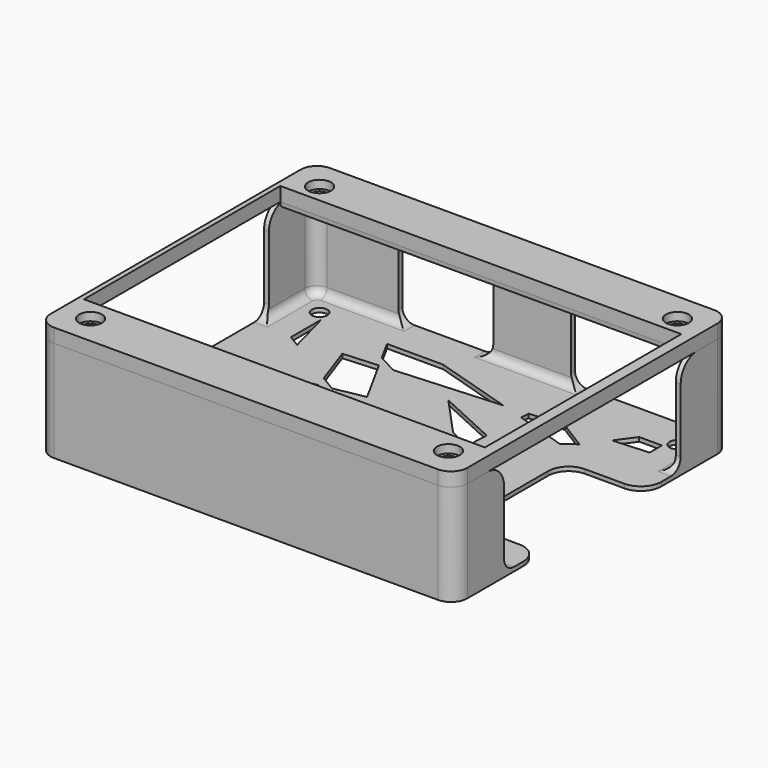
from build123d import *

# Parameters (mm, degrees)
F1_W      = 101.8573045731
F1_H      = 84.3658432415
F1_W_2    = 99.4573066576
F1_H_2    = 81.9658453261
F2_DEPTH  = 1
F3_DEPTH  = 23.7
F4_W      = 54
F4_H      = 23.7
F5_DEPTH  = 101.8583045731
F7_DEPTH  = 25
F0_R      = 1.9
F8_DEPTH  = 25
F9_R      = 3
F10_R     = 4
F11_R     = 3
F12_R     = 5
F14_DEPTH = 25
F15_R     = 5
F17_R     = 1.9
F18_DEPTH = 3.4
F19_DEPTH = 1
F19_TAPER = 4
F20_R     = 2.8028286172
F20_R_2   = 1.9
F21_DEPTH = 2
F23_DEPTH = 25
F24_R     = 2


with BuildPart() as f2:
    # F1 (on Top) → F2 (new body)
    with BuildSketch(Plane.XY):
        Rectangle(F1_W, F1_H)
        Rectangle(F1_W_2, F1_H_2, mode=Mode.SUBTRACT)
        Rectangle(F1_W_2, F1_H_2)
    extrude(amount=-F2_DEPTH)

    # F1 (on Top) → F3 (join)
    with BuildSketch(Plane.XY):
        Rectangle(F1_W, F1_H)
        Rectangle(F1_W_2, F1_H_2, mode=Mode.SUBTRACT)
    extrude(amount=F3_DEPTH)

    # F4 (on face) → F5 (cut, through all)
    with BuildSketch(Plane(origin=(-50.9286522865, 0, 0), x_dir=(0, -1, 0), z_dir=(-1, 0, 0))):
        with Locations((0, 11.85)):
            Rectangle(F4_W, F4_H)
    extrude(amount=-F5_DEPTH, mode=Mode.SUBTRACT)

    # F6 (on face) → F7 (cut)
    with BuildSketch(Plane(origin=(0, 42.1829216208, 0), x_dir=(-1, 0, 0), z_dir=(0, 1, 0))):
        Polygon((-12.9286522865, 0), (-12.9286522865, 11.35), (-12.9286522865, 25.37307702), (-44.0330952406, 25.37307702), (-44.0330952406, 0), align=None)
        Polygon((6.0713477135, 25.847222656), (6.0713477135, 7.5958021916), (6.0713477135, 0), (29.2794182897, 0), (29.2794182897, 25.847222656), align=None)
    extrude(amount=-F7_DEPTH, mode=Mode.SUBTRACT)

    # F0 (on Top) → F8 (cut)
    with BuildSketch(Plane.XY):
        with Locations((43.7286533288, 34.982922663)):
            Circle(F0_R)
        with Locations((43.7286533288, -34.982922663)):
            Circle(F0_R)
        with Locations((-43.7286533288, 34.982922663)):
            Circle(F0_R)
        with Locations((-43.7286533288, -34.982922663)):
            Circle(F0_R)
    extrude(amount=-F8_DEPTH, mode=Mode.SUBTRACT)

    # F9
    f9_edges = [f2.edges().sort_by_distance(p)[0] for p in [
        (49.728653, -40.982923, 11.85),
        (-49.728653, -40.982923, 11.85),
        (-49.728653, 40.982923, 11.85),
        (49.728653, 40.982923, 11.85),
    ]]
    fillet(f9_edges, radius=F9_R)

    # F10
    f10_edges = [f2.edges().sort_by_distance(p)[0] for p in [
        (-50.928652, 42.182922, 11.35),
        (-50.928652, -42.182922, 11.35),
        (50.928652, -42.182922, 11.35),
        (50.928652, 42.182922, 11.35),
    ]]
    fillet(f10_edges, radius=F10_R)

    # F11
    f11_edges = [f2.edges().sort_by_distance(p)[0] for p in [
        (-50.328653, 27, 0),
        (-29.279418, 41.582922, 0),
        (-6.071348, 41.582922, 0),
        (12.928652, 41.582922, 0),
        (44.033095, 41.582922, 0),
        (50.328653, 27, 0),
        (50.328653, -27, 0),
        (-50.328653, -27, 0),
    ]]
    fillet(f11_edges, radius=F11_R)

    # F12
    f12_edges = [f2.edges().sort_by_distance(p)[0] for p in [
        (50.328653, -27, 23.7),
        (50.328653, 27, 23.7),
        (44.033095, 41.582922, 23.7),
        (12.928652, 41.582922, 23.7),
        (-6.071348, 41.582922, 23.7),
        (-29.279418, 41.582922, 23.7),
        (-50.328653, 27, 23.7),
        (-50.328653, -27, 23.7),
    ]]
    fillet(f12_edges, radius=F12_R)

    # F13 (on face) → F14 (cut)
    with BuildSketch(Plane(origin=(0, 0, -1), x_dir=(1, 0, 0), z_dir=(0, 0, -1))):
        Polygon((50.9286522865, 0), (50.9286522865, 16.0555634648), (31.2976017594, 16.0555634648), (31.2976017594, 0), (31.2976017594, -16.0555634648), (50.9286522865, -16.0555634648), align=None)
    extrude(amount=-F14_DEPTH, mode=Mode.SUBTRACT)

    # F15
    f15_edges = [f2.edges().sort_by_distance(p)[0] for p in [
        (50.928652, -16.055563, -0.5),
        (50.928652, 16.055563, -0.5),
        (31.297602, -16.055563, -0.5),
        (31.297602, 16.055563, -0.5),
    ]]
    fillet(f15_edges, radius=F15_R)

    # F22 (on face) → F23 (cut)
    with BuildSketch(Plane(origin=(0, 0, -1), x_dir=(1, 0, 0), z_dir=(0, 0, -1))):
        Polygon((-29.4763375006, 14.8269218376), (-41.6286520634, 12.3842693865), (-30.3887994705, 9.3961659471), (-29.0076859915, 14.5912712147), align=None)
        Polygon((-10.8715390327, 29.0833591801), (-15.9313136106, 27.743293622), (-12.1721135632, 25.3909763414), align=None)
        Polygon((-24.1448692977, 32.8829213977), (-41.6286520634, 32.8829213977), (-41.6286520634, 20.9374334663), (-26.2368387197, 25.013907353), align=None)
        Polygon((-15.6970236635, 15.3836163194), (-20.9847782869, 10.5571367647), (-17.9368811333, 9.0245718443), align=None)
        Polygon((-32.9943795181, -0.4048119131), (-35.4038891191, -9.468264128), (-25.1375269952, -11.4183482529), (-18.8833677873, 6.3374585753), (-24.0909853022, 7.7218984226), align=None)
        Polygon((-26.1431570385, -14.2733719574), (-29.7097056452, -24.3989453556), (-21.2132293912, -24.9611379018), (-14.8402038289, -13.3743133936), (-22.301487185, -11.9570508766), align=None)
        Polygon((-5.5360004898, 2.789074484), (-5.8971521934, 2.885086299), (-9.9716865757, -4.5228417533), (-1.342161859, 0.6802992716), align=None)
        Polygon((-22.7277484281, -27.7146913158), (-25.5703963339, -32.8829213977), (-9.9331525483, -25.70751498), (-17.8456036869, -25.18396605), align=None)
        Polygon((-39.206147282, -23.77058737), (-41.6286520634, -23.6102957278), (-41.6286520634, -32.8829213977), align=None)
        Polygon((-38.6929646651, -21.840233524), (-41.6286520634, -23.6102957278), (-39.206147282, -23.77058737), align=None)
        Polygon((-9.9331525483, -25.70751498), (-25.5703963339, -32.8829213977), (-11.849696748, -32.8829213977), (-5.5335982145, -25.9986235031), align=None)
        Polygon((-5.5335982145, -25.9986235031), (-11.849696748, -32.8829213977), (7.6651824891, -26.8719568602), align=None)
        Polygon((2.9486668234, -16.7532896893), (-1.8734205455, -22.0091744329), (7.6390471274, -17.6442222378), align=None)
        Polygon((7.0570029567, -12.2753655968), (2.9486668234, -16.7532896893), (7.6390471274, -17.6442222378), (12.9477911078, -15.2082177764), (12.6630292841, -9.3694065932), align=None)
        with BuildLine():
            Line((13.4300364537, -25.0962690722), (13.5355816391, -27.2603878458))
            Line((13.5355816391, -27.2603878458), (21.9606679178, -27.8178566794))
            Line((21.9606679178, -27.8178566794), (29.0744918276, -23.3972282347))
            ThreePointArc((29.0744918276, -23.3972282347), (27.5588064071, -22.3747269573), (26.1859746307, -21.1671905935))
            Line((26.1859746307, -21.1671905935), (13.4300364537, -25.0962690722))
        make_face()
        Polygon((32.8745938929, -28.5400063859), (36.0836610198, -32.8829213977), (41.6286520634, -29.1192425428), align=None)
        Polygon((41.6286520634, -29.1192425428), (36.0836610198, -32.8829213977), (41.6286520634, -32.8829213977), align=None)
        Polygon((1.7053230027, 16.7071783437), (4.4184203361, 21.6398719863), (-3.6014076253, 20.0278620004), align=None)
        Polygon((11.0853349082, 22.9799422369), (4.4184203361, 21.6398719863), (1.7053230027, 16.7071783437), (11.6961624804, 10.4554162521), align=None)
        Polygon((27.8325551851, 26.3461848112), (15.948086977, 32.8829213977), (19.0470213151, 24.5802655922), align=None)
        with BuildLine():
            ThreePointArc((21.9976015364, 11.0555634648), (22.1447687516, 13.1018587106), (22.5832412801, 15.1060354155))
            Line((22.5832412801, 15.1060354155), (13.2536724335, 9.4808052893))
            Line((13.2536724335, 9.4808052893), (21.9976015364, 4.0092966519))
            Line((21.9976015364, 4.0092966519), (21.9976015364, 11.0555634648))
        make_face()
        Polygon((21.9976015364, -11.0555634648), (21.9976015364, -4.5307057564), (15.6081391182, -7.8427693747), align=None)
        Polygon((15.6987796861, -2.8561703406), (12.3013253975, -1.9529605555), (12.5126636537, -6.286280796), (12.539428152, -6.2997387079), align=None)
        Polygon((-32.9943795181, -0.4048119131), (-41.6286520634, -8.2858772948), (-35.4038891191, -9.468264128), align=None)
        Polygon((41.6286520634, 32.8829213977), (30.8725539127, 32.8829213977), (41.6286520634, 29.1192425428), align=None)
    extrude(amount=-F23_DEPTH, mode=Mode.SUBTRACT)

    # F24
    f24_edges = [f2.edges().sort_by_distance(p)[0] for p in [
        (0, -40.982923, 0),
        (48.849974, -40.104243, 0),
        (49.728653, -30.991461, 0),
        (-48.849974, -40.104243, 0),
        (-49.728653, -30.991461, 0),
        (-49.728653, 30.991461, 0),
        (-48.849974, 40.104243, 0),
        (-36.504036, 40.982923, 0),
        (3.428652, 40.982923, 0),
        (43.880874, 40.982923, 0),
        (48.849974, 40.104243, 0),
        (49.728653, 30.991461, 0),
    ]]
    fillet(f24_edges, radius=F24_R)


with BuildPart() as f18:
    # F17 (on offset) → F18 (new body)
    with BuildSketch(Plane.XY.offset(23.7)):
        with BuildLine():
            Line((50.9286522865, -38.1829216208), (50.9286522865, -32))
            Line((50.9286522865, -32), (50.9286522865, 27))
            Line((50.9286522865, 27), (50.9286522865, 32))
            Line((50.9286522865, 32), (50.9286522865, 38.1829216208))
            ThreePointArc((50.9286522865, 38.1829216208), (50.4227739084, 40.1299999684), (49.0330952406, 41.5845858977))
            ThreePointArc((49.0330952406, 41.5845858977), (48.0225770765, 42.030431017), (46.9286522865, 42.1829216208))
            Line((46.9286522865, 42.1829216208), (44.0330952406, 42.1829216208))
            Line((44.0330952406, 42.1829216208), (-34.2794182897, 42.1829216208))
            Line((-34.2794182897, 42.1829216208), (-46.9286522865, 42.1829216208))
            ThreePointArc((-46.9286522865, 42.1829216208), (-49.7570794113, 41.0113487455), (-50.9286522865, 38.1829216208))
            Line((-50.9286522865, 38.1829216208), (-50.9286522865, 32))
            Line((-50.9286522865, 32), (-50.9286522865, -32))
            Line((-50.9286522865, -32), (-50.9286522865, -38.1829216208))
            ThreePointArc((-50.9286522865, -38.1829216208), (-49.7570794113, -41.0113487455), (-46.9286522865, -42.1829216208))
            Line((-46.9286522865, -42.1829216208), (46.9286522865, -42.1829216208))
            ThreePointArc((46.9286522865, -42.1829216208), (49.7570794113, -41.0113487455), (50.9286522865, -38.1829216208))
        make_face()
        with BuildLine():
            ThreePointArc((-46.7286533288, -40.982922663), (-48.8499736724, -40.1042430066), (-49.7286533288, -37.982922663))
            Line((-49.7286533288, -37.982922663), (-49.7286533288, -32))
            Line((-49.7286533288, -32), (-49.7286533288, -29.517077337))
            Line((-49.7286533288, -29.517077337), (-49.7286533288, 30.482922663))
            Line((-49.7286533288, 30.482922663), (-49.7286533288, 32))
            Line((-49.7286533288, 32), (-49.7286533288, 37.982922663))
            ThreePointArc((-49.7286533288, 37.982922663), (-48.8499736724, 40.1042430066), (-46.7286533288, 40.982922663))
            Line((-46.7286533288, 40.982922663), (-34.2794182897, 40.982922663))
            Line((-34.2794182897, 40.982922663), (44.0330952406, 40.982922663))
            Line((44.0330952406, 40.982922663), (46.7286533288, 40.982922663))
            ThreePointArc((46.7286533288, 40.982922663), (48.00096256, 40.6997644362), (49.0330952406, 39.9037421432))
            ThreePointArc((49.0330952406, 39.9037421432), (49.5494090551, 39.0043614191), (49.7286533288, 37.982922663))
            Line((49.7286533288, 37.982922663), (49.7286533288, 32))
            Line((49.7286533288, 32), (49.7286533288, 27))
            Line((49.7286533288, 27), (49.7286533288, -32))
            Line((49.7286533288, -32), (49.7286533288, -37.982922663))
            ThreePointArc((49.7286533288, -37.982922663), (48.8499736724, -40.1042430066), (46.7286533288, -40.982922663))
            Line((46.7286533288, -40.982922663), (-46.7286533288, -40.982922663))
        make_face(mode=Mode.SUBTRACT)
        with BuildLine():
            Line((-49.7286533288, -32), (-49.7286533288, -37.982922663))
            ThreePointArc((-49.7286533288, -37.982922663), (-48.8499736724, -40.1042430066), (-46.7286533288, -40.982922663))
            Line((-46.7286533288, -40.982922663), (46.7286533288, -40.982922663))
            ThreePointArc((46.7286533288, -40.982922663), (48.8499736724, -40.1042430066), (49.7286533288, -37.982922663))
            Line((49.7286533288, -37.982922663), (49.7286533288, -32))
            Line((49.7286533288, -32), (49.7286533288, 27))
            Line((49.7286533288, 27), (49.7286533288, 32))
            Line((49.7286533288, 32), (49.7286533288, 37.982922663))
            ThreePointArc((49.7286533288, 37.982922663), (49.5494090551, 39.0043614191), (49.0330952406, 39.9037421432))
            ThreePointArc((49.0330952406, 39.9037421432), (48.00096256, 40.6997644362), (46.7286533288, 40.982922663))
            Line((46.7286533288, 40.982922663), (44.0330952406, 40.982922663))
            Line((44.0330952406, 40.982922663), (-34.2794182897, 40.982922663))
            Line((-34.2794182897, 40.982922663), (-46.7286533288, 40.982922663))
            ThreePointArc((-46.7286533288, 40.982922663), (-48.8499736724, 40.1042430066), (-49.7286533288, 37.982922663))
            Line((-49.7286533288, 37.982922663), (-49.7286533288, 32))
            Line((-49.7286533288, 32), (-49.7286533288, 30.482922663))
            Line((-49.7286533288, 30.482922663), (48.2879653573, 30.482922663))
            Line((48.2879653573, 30.482922663), (48.2879653573, -29.517077337))
            Line((48.2879653573, -29.517077337), (-49.7286533288, -29.517077337))
            Line((-49.7286533288, -29.517077337), (-49.7286533288, -32))
        make_face()
        with Locations((-43.7286533288, -34.982922663)):
            Circle(F17_R, mode=Mode.SUBTRACT)
        with Locations((43.7286533288, -34.982922663)):
            Circle(F17_R, mode=Mode.SUBTRACT)
        with Locations((-43.7286533288, 34.982922663)):
            Circle(F17_R, mode=Mode.SUBTRACT)
        with Locations((43.7286533288, 34.982922663)):
            Circle(F17_R, mode=Mode.SUBTRACT)
    extrude(amount=F18_DEPTH)

    # F17 (on offset) → F19 (join)
    with BuildSketch(Plane.XY.offset(23.7)):
        with BuildLine():
            Line((-49.7286533288, -32), (-49.7286533288, -37.982922663))
            ThreePointArc((-49.7286533288, -37.982922663), (-48.8499736724, -40.1042430066), (-46.7286533288, -40.982922663))
            Line((-46.7286533288, -40.982922663), (46.7286533288, -40.982922663))
            ThreePointArc((46.7286533288, -40.982922663), (48.8499736724, -40.1042430066), (49.7286533288, -37.982922663))
            Line((49.7286533288, -37.982922663), (49.7286533288, -32))
            Line((49.7286533288, -32), (49.7286533288, 27))
            Line((49.7286533288, 27), (49.7286533288, 32))
            Line((49.7286533288, 32), (49.7286533288, 37.982922663))
            ThreePointArc((49.7286533288, 37.982922663), (49.5494090551, 39.0043614191), (49.0330952406, 39.9037421432))
            ThreePointArc((49.0330952406, 39.9037421432), (48.00096256, 40.6997644362), (46.7286533288, 40.982922663))
            Line((46.7286533288, 40.982922663), (44.0330952406, 40.982922663))
            Line((44.0330952406, 40.982922663), (-34.2794182897, 40.982922663))
            Line((-34.2794182897, 40.982922663), (-46.7286533288, 40.982922663))
            ThreePointArc((-46.7286533288, 40.982922663), (-48.8499736724, 40.1042430066), (-49.7286533288, 37.982922663))
            Line((-49.7286533288, 37.982922663), (-49.7286533288, 32))
            Line((-49.7286533288, 32), (-49.7286533288, 30.482922663))
            Line((-49.7286533288, 30.482922663), (48.2879653573, 30.482922663))
            Line((48.2879653573, 30.482922663), (48.2879653573, -29.517077337))
            Line((48.2879653573, -29.517077337), (-49.7286533288, -29.517077337))
            Line((-49.7286533288, -29.517077337), (-49.7286533288, -32))
        make_face()
        with Locations((-43.7286533288, -34.982922663)):
            Circle(F17_R, mode=Mode.SUBTRACT)
        with Locations((43.7286533288, -34.982922663)):
            Circle(F17_R, mode=Mode.SUBTRACT)
        with Locations((-43.7286533288, 34.982922663)):
            Circle(F17_R, mode=Mode.SUBTRACT)
        with Locations((43.7286533288, 34.982922663)):
            Circle(F17_R, mode=Mode.SUBTRACT)
    extrude(amount=-F19_DEPTH, taper=F19_TAPER)

    # F20 (on face) → F21 (cut)
    with BuildSketch(Plane.XY.offset(27.1)):
        with Locations((-43.7286533288, 34.982922663)):
            Circle(F20_R)
        with Locations((-43.7286533288, 34.982922663)):
            Circle(F20_R_2, mode=Mode.SUBTRACT)
        with Locations((43.7286533288, 34.982922663)):
            Circle(F20_R)
        with Locations((43.7286533288, 34.982922663)):
            Circle(F20_R_2, mode=Mode.SUBTRACT)
        with Locations((43.7286533288, -34.982922663)):
            Circle(F20_R)
        with Locations((43.7286533288, -34.982922663)):
            Circle(F20_R_2, mode=Mode.SUBTRACT)
        with Locations((-43.7286533288, -34.982922663)):
            Circle(F20_R)
        with Locations((-43.7286533288, -34.982922663)):
            Circle(F20_R_2, mode=Mode.SUBTRACT)
    extrude(amount=-F21_DEPTH, mode=Mode.SUBTRACT)


solid = Compound([f2.part, f18.part])
